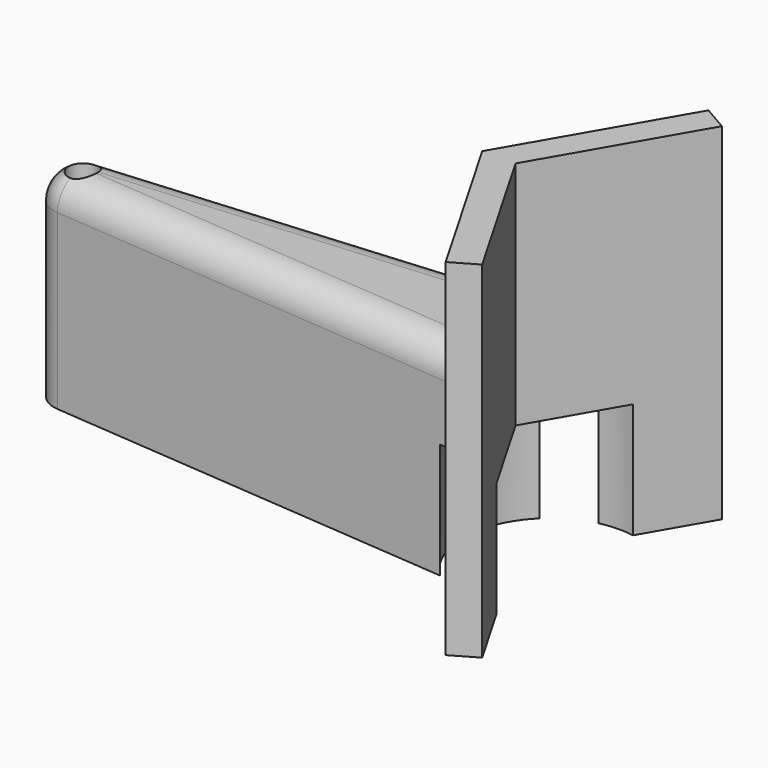
from build123d import *

# Parameters (mm, degrees)
F0_R         = 2.5
F1_DEPTH     = 35
F3_DEPTH     = 25
F4_T4_DEPTH  = 88.824838337
F4_T9_DEPTH  = 88.824838337
F4_T12_ANGLE = 170.716427301
F5_R         = 15
F6_DEPTH     = 20


# Not quite as in the source:
# - a fillet or chamfer that OpenCascade refuses, or shapes differently, is made with other operations: its cross-section is extruded or revolved along the edge and cut away or added


with BuildPart() as f1:
    # F0 (on Top) → F1 (new body)
    with BuildSketch(Plane.XY):
        with BuildLine():
            Line((0.6698729811, 11.1602540378), (-75.4046293156, 4.9836006177))
            ThreePointArc((-75.4046293156, 4.9836006177), (-80, 0), (-75.4046293156, -4.9836006177))
            Line((-75.4046293156, -4.9836006177), (0.6698729811, -11.1602540378))
            Line((0.6698729811, -11.1602540378), (10.6698729811, -28.4807621135))
            Line((10.6698729811, -28.4807621135), (15, -25.9807621135))
            Line((15, -25.9807621135), (0, 0))
            Line((0, 0), (15, 25.9807621135))
            Line((15, 25.9807621135), (10.6698729811, 28.4807621135))
            Line((10.6698729811, 28.4807621135), (0.6698729811, 11.1602540378))
        make_face()
        with Locations((-75, 0)):
            Circle(F0_R, mode=Mode.SUBTRACT)
    extrude(amount=F1_DEPTH)

    # F2 (on face) → F3 (join)
    with BuildSketch(Plane.XY.offset(35)):
        Polygon((15, -25.9807621135), (0, 0), (15, 25.9807621135), (10.6698729811, 28.4807621135), (0.6698729811, 11.1602540378), (-5.7735026919, 0), (0.6698729811, -11.1602540378), (10.6698729811, -28.4807621135), align=None)
    extrude(amount=F3_DEPTH)

    # F4: fillet of radius 5 on 2 edges, made by hand


with BuildPart() as f4_tool2:
    # F4_s3 → F4_t4 (new body)
    with BuildSketch(Plane(origin=(-74.5088253508, 6.0495327217, 0), x_dir=(0, 0, 1), z_dir=(0.9967201235, -0.0809258631, 0))):
        with BuildLine():
            ThreePointArc((35, 6.0694397342), (33.5355339059, 9.6049736401), (30, 11.0694397342))
            Line((30, 11.0694397342), (35, 11.0694397342))
            Line((35, 11.0694397342), (35, 6.0694397342))
        make_face()
    extrude(amount=F4_T4_DEPTH)

    split(bisect_by=Plane(origin=(-4.3301270189, -2.5, 0), x_dir=(0, 0, 1), z_dir=(-0.8660254038, -0.5, 0)), keep=Keep.TOP)


with BuildPart() as f1_1:
    add(f1.part)

    # F4_t1: cut F4_tool2
    add(f4_tool2.part, mode=Mode.SUBTRACT)


with BuildPart() as f4_tool7:
    # F4_s8 → F4_t9 (new body)
    with BuildSketch(Plane(origin=(14.0246784902, 1.1386939874, 0), x_dir=(0, 0, 1), z_dir=(-0.9967201235, -0.0809258631, 0))):
        with BuildLine():
            ThreePointArc((30, 11.0694397342), (33.5355339059, 9.6049736401), (35, 6.0694397342))
            Line((35, 6.0694397342), (35, 11.0694397342))
            Line((35, 11.0694397342), (30, 11.0694397342))
        make_face()
    extrude(amount=F4_T9_DEPTH)

    split(bisect_by=Plane(origin=(-4.3301270189, 2.5, 0), x_dir=(0, 0, 1), z_dir=(-0.8660254038, 0.5, 0)), keep=Keep.TOP)


with BuildPart() as f1_2:
    add(f1_1.part)

    # F4_t6: cut F4_tool7
    add(f4_tool7.part, mode=Mode.SUBTRACT)

    # F4_s11 → F4_t12 (revolve, cut)
    with BuildSketch(Plane(origin=(-74.5088253508, -6.0495327217, 0), x_dir=(0, 0, 1), z_dir=(0.9967201235, 0.0809258631, 0))):
        with BuildLine():
            ThreePointArc((35, -6.0694397342), (33.5355339059, -9.6049736401), (30, -11.0694397342))
            Line((30, -11.0694397342), (35, -11.0694397342))
            Line((35, -11.0694397342), (35, -6.0694397342))
        make_face()
    revolve(axis=Axis((-75, 0, 35), (0, 0, 1)), revolution_arc=F4_T12_ANGLE, mode=Mode.SUBTRACT)

    # F5 (on Top) → F6 (cut)
    with BuildSketch(Plane.XY):
        with Locations((6, 0)):
            Circle(F5_R)
    extrude(amount=F6_DEPTH, mode=Mode.SUBTRACT)


solid = f1_2.part
